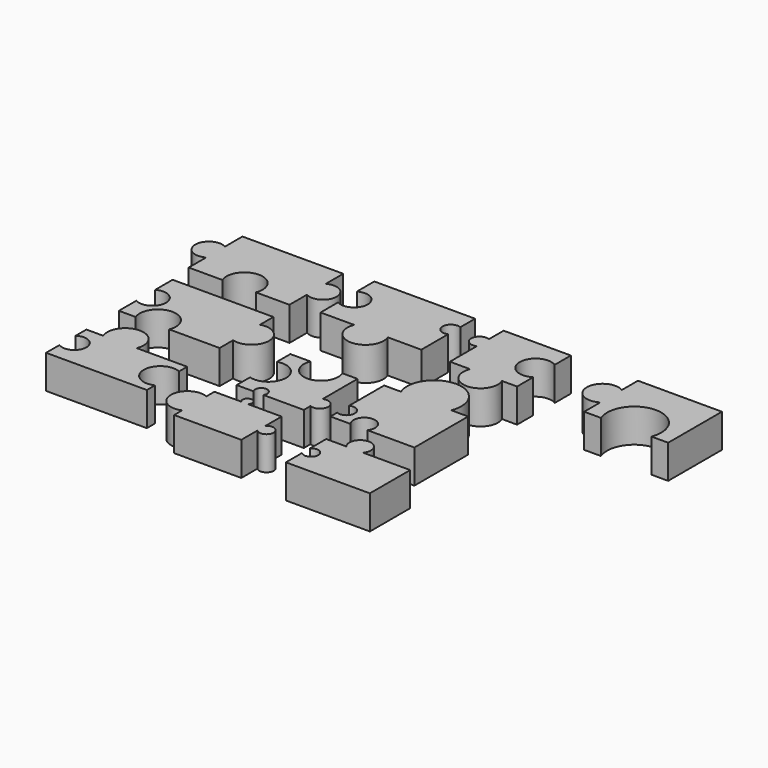
from build123d import *

# Parameters (mm, degrees)
F1_DEPTH  = 25.4
F3_DEPTH  = 25.4
F5_DEPTH  = 25.4
F7_DEPTH  = 25.4
F9_DEPTH  = 25.4
F11_DEPTH = 25.4
F13_DEPTH = 25.4
F15_DEPTH = 25.4
F17_DEPTH = 25.4
F19_DEPTH = 25.4


# Not quite as in the source:
# - a feature names something its author has since deleted; it is built from what else it names


with BuildPart() as f1:
    # F0 (on Top) → F1 (new body)
    with BuildSketch(Plane.XY):
        with BuildLine():
            Line((-78.5367997915, 29.1591999254), (-78.5367997915, 46.9391999254))
            ThreePointArc((-78.5367997915, 46.9391999254), (-93.8558671318, 38.0491999254), (-78.5367997915, 29.1591999254))
        make_face()
        with BuildLine():
            Line((-2.3367997915, 63.4491999254), (-78.5367997915, 63.4491999254))
            Line((-78.5367997915, 63.4491999254), (-78.5367997915, 46.9391999254))
            Line((-78.5367997915, 46.9391999254), (-78.5367997915, 29.1591999254))
            Line((-78.5367997915, 29.1591999254), (-78.5367997915, 12.6491999254))
            Line((-78.5367997915, 12.6491999254), (-53.1367997915, 12.6491999254))
            ThreePointArc((-53.1367997915, 12.6491999254), (-40.4367997915, 31.4075185355), (-27.7367997915, 12.6491999254))
            Line((-27.7367997915, 12.6491999254), (-2.3367997915, 12.6491999254))
            Line((-2.3367997915, 12.6491999254), (-2.3367997915, 29.1591999254))
            Line((-2.3367997915, 29.1591999254), (-2.3367997915, 46.9391999254))
            Line((-2.3367997915, 46.9391999254), (-2.3367997915, 63.4491999254))
        make_face()
        with BuildLine():
            ThreePointArc((-2.3367997915, 29.1591999254), (12.9822675489, 38.0491999254), (-2.3367997915, 46.9391999254))
            Line((-2.3367997915, 46.9391999254), (-2.3367997915, 29.1591999254))
        make_face()
    extrude(amount=F1_DEPTH)


with BuildPart() as f3:
    # F2 (on Top) → F3 (new body)
    with BuildSketch(Plane.XY):
        with BuildLine():
            Line((68.946869266, 16.4046303093), (43.546869266, 16.4046303093))
            ThreePointArc((43.546869266, 16.4046303093), (56.246869266, -2.3536883008), (68.946869266, 16.4046303093))
        make_face()
        with BuildLine():
            Line((94.346869266, 67.2046303093), (18.146869266, 67.2046303093))
            Line((18.146869266, 67.2046303093), (18.146869266, 50.6946303093))
            ThreePointArc((18.146869266, 50.6946303093), (33.4659366064, 41.8046303093), (18.146869266, 32.9146303093))
            Line((18.146869266, 32.9146303093), (18.146869266, 16.4046303093))
            Line((18.146869266, 16.4046303093), (43.546869266, 16.4046303093))
            Line((43.546869266, 16.4046303093), (68.946869266, 16.4046303093))
            Line((68.946869266, 16.4046303093), (94.346869266, 16.4046303093))
            Line((94.346869266, 16.4046303093), (94.346869266, 41.8046303093))
            ThreePointArc((94.346869266, 41.8046303093), (85.5528445619, 47.5196303093), (94.346869266, 53.2346303093))
            Line((94.346869266, 53.2346303093), (94.346869266, 67.2046303093))
        make_face()
    extrude(amount=F3_DEPTH)


with BuildPart() as f5:
    # F4 (on Top) → F5 (new body)
    with BuildSketch(Plane.XY):
        with BuildLine():
            Line((-50.8, -5.4863997316), (-76.2, -5.4863997316))
            Line((-76.2, -5.4863997316), (-76.2, -21.9963997316))
            ThreePointArc((-76.2, -21.9963997316), (-60.8809326597, -30.8863997316), (-76.2, -39.7763997316))
            Line((-76.2, -39.7763997316), (-76.2, -56.2863997316))
            Line((-76.2, -56.2863997316), (-63.5, -56.2863997316))
            ThreePointArc((-63.5, -56.2863997316), (-50.8, -37.5280811215), (-38.1, -56.2863997316))
            Line((-38.1, -56.2863997316), (0, -56.2863997316))
            Line((0, -56.2863997316), (0, -43.5863997316))
            Line((0, -43.5863997316), (0, -18.1863997316))
            Line((0, -18.1863997316), (0, -5.4863997316))
            Line((0, -5.4863997316), (-25.4, -5.4863997316))
            ThreePointArc((-25.4, -5.4863997316), (-38.1, -24.2447183418), (-50.8, -5.4863997316))
        make_face()
        with BuildLine():
            Line((-25.4, -5.4863997316), (-50.8, -5.4863997316))
            ThreePointArc((-50.8, -5.4863997316), (-38.1, -24.2447183418), (-25.4, -5.4863997316))
        make_face()
        with BuildLine():
            ThreePointArc((0, -43.5863997316), (17.0691892663, -30.8863997316), (0, -18.1863997316))
            Line((0, -18.1863997316), (0, -43.5863997316))
        make_face()
    extrude(amount=F5_DEPTH)


with BuildPart() as f7:
    # F6 (on Top) → F7 (new body)
    with BuildSketch(Plane.XY):
        with BuildLine():
            ThreePointArc((88.2271643072, -80.6943764091), (97.0211890114, -74.9793764091), (88.2271643072, -69.2643764091))
            Line((88.2271643072, -69.2643764091), (88.2271643072, -80.6943764091))
        make_face()
        with BuildLine():
            Line((52.6671643072, -36.2443764091), (37.4271643072, -36.2443764091))
            Line((37.4271643072, -36.2443764091), (37.4271643072, -48.9443764091))
            ThreePointArc((37.4271643072, -48.9443764091), (54.4963535736, -61.6443764091), (37.4271643072, -74.3443764091))
            Line((37.4271643072, -74.3443764091), (37.4271643072, -87.0443764091))
            Line((37.4271643072, -87.0443764091), (50.1271643072, -87.0443764091))
            ThreePointArc((50.1271643072, -87.0443764091), (53.9371643072, -79.9253262892), (57.7471643072, -87.0443764091))
            Line((57.7471643072, -87.0443764091), (88.2271643072, -87.0443764091))
            Line((88.2271643072, -87.0443764091), (88.2271643072, -80.6943764091))
            Line((88.2271643072, -80.6943764091), (88.2271643072, -69.2643764091))
            Line((88.2271643072, -69.2643764091), (88.2271643072, -36.2443764091))
            Line((88.2271643072, -36.2443764091), (76.7971643072, -36.2443764091))
            ThreePointArc((76.7971643072, -36.2443764091), (64.7321643072, -54.4152367704), (52.6671643072, -36.2443764091))
        make_face()
    extrude(amount=F7_DEPTH)


with BuildPart() as f9:
    # F8 (on Top) → F9 (new body)
    with BuildSketch(Plane.XY):
        with BuildLine():
            Line((117.092727313, 40.3700199814), (117.092727313, 14.9700199814))
            Line((117.092727313, 14.9700199814), (132.332727313, 14.9700199814))
            Line((132.332727313, 14.9700199814), (156.462727313, 14.9700199814))
            Line((156.462727313, 14.9700199814), (167.892727313, 14.9700199814))
            Line((167.892727313, 14.9700199814), (167.892727313, 30.2100199814))
            ThreePointArc((167.892727313, 30.2100199814), (149.5615712753, 40.3700199814), (167.892727313, 50.5300199814))
            Line((167.892727313, 50.5300199814), (167.892727313, 65.7700199814))
            Line((167.892727313, 65.7700199814), (117.092727313, 65.7700199814))
            Line((117.092727313, 65.7700199814), (117.092727313, 51.8000199814))
            Line((117.092727313, 51.8000199814), (117.092727313, 40.3700199814))
        make_face()
        with BuildLine():
            Line((156.462727313, 14.9700199814), (132.332727313, 14.9700199814))
            ThreePointArc((132.332727313, 14.9700199814), (144.397727313, -3.2008403799), (156.462727313, 14.9700199814))
        make_face()
        with BuildLine():
            ThreePointArc((117.092727313, 51.8000199814), (108.2987026089, 46.0850199814), (117.092727313, 40.3700199814))
            Line((117.092727313, 40.3700199814), (117.092727313, 51.8000199814))
        make_face()
    extrude(amount=F9_DEPTH)


with BuildPart() as f11:
    # F10 (on Top) → F11 (new body)
    with BuildSketch(Plane.XY):
        with BuildLine():
            Line((218.9528409719, 29.8046059906), (218.9528409719, 50.1246059906))
            ThreePointArc((218.9528409719, 50.1246059906), (200.6216849342, 39.9646059906), (218.9528409719, 29.8046059906))
        make_face()
        with BuildLine():
            Line((282.4528409719, 65.3646059906), (218.9528409719, 65.3646059906))
            Line((218.9528409719, 65.3646059906), (218.9528409719, 50.1246059906))
            Line((218.9528409719, 50.1246059906), (218.9528409719, 29.8046059906))
            Line((218.9528409719, 29.8046059906), (218.9528409719, 14.5646059906))
            Line((218.9528409719, 14.5646059906), (231.6528409719, 14.5646059906))
            ThreePointArc((231.6528409719, 14.5646059906), (250.7028409719, 42.7020839058), (269.7528409719, 14.5646059906))
            Line((269.7528409719, 14.5646059906), (282.4528409719, 14.5646059906))
            Line((282.4528409719, 14.5646059906), (282.4528409719, 65.3646059906))
        make_face()
    extrude(amount=F11_DEPTH)


with BuildPart() as f13:
    # F12 (on Top) → F13 (new body)
    with BuildSketch(Plane.XY):
        with BuildLine():
            ThreePointArc((156.5685857674, -33.0217852473), (137.5185857674, -4.8843073321), (118.4685857674, -33.0217852473))
            Line((118.4685857674, -33.0217852473), (156.5685857674, -33.0217852473))
        make_face()
        with BuildLine():
            Line((118.4685857674, -33.0217852473), (105.7685857674, -33.0217852473))
            Line((105.7685857674, -33.0217852473), (105.7685857674, -66.0417852473))
            ThreePointArc((105.7685857674, -66.0417852473), (114.5626104715, -71.7567852473), (105.7685857674, -77.4717852473))
            Line((105.7685857674, -77.4717852473), (105.7685857674, -83.8217852473))
            Line((105.7685857674, -83.8217852473), (121.0085857674, -83.8217852473))
            ThreePointArc((121.0085857674, -83.8217852473), (127.3585857674, -70.6098174658), (133.7085857674, -83.8217852473))
            Line((133.7085857674, -83.8217852473), (169.2685857674, -83.8217852473))
            Line((169.2685857674, -83.8217852473), (169.2685857674, -33.0217852473))
            Line((169.2685857674, -33.0217852473), (156.5685857674, -33.0217852473))
            Line((156.5685857674, -33.0217852473), (118.4685857674, -33.0217852473))
        make_face()
    extrude(amount=F13_DEPTH)


with BuildPart() as f15:
    # F14 (on Top) → F15 (new body)
    with BuildSketch(Plane.XY):
        with BuildLine():
            ThreePointArc((-38.1, -86.9720183969), (-50.8, -68.2136997867), (-63.5, -86.9720183969))
            Line((-63.5, -86.9720183969), (-38.1, -86.9720183969))
        make_face()
        with BuildLine():
            Line((-63.5, -86.9720183969), (-76.2, -86.9720183969))
            Line((-76.2, -86.9720183969), (-76.2, -97.1320183969))
            ThreePointArc((-76.2, -97.1320183969), (-61.9618997603, -104.7520183969), (-76.2, -112.3720183969))
            Line((-76.2, -112.3720183969), (-76.2, -125.0720183969))
            Line((-76.2, -125.0720183969), (0, -125.0720183969))
            Line((0, -125.0720183969), (0, -117.4520183969))
            ThreePointArc((0, -117.4520183969), (-17.5880494083, -106.0220183969), (0, -94.5920183969))
            Line((0, -94.5920183969), (0, -86.9720183969))
            Line((0, -86.9720183969), (-38.1, -86.9720183969))
            Line((-38.1, -86.9720183969), (-63.5, -86.9720183969))
        make_face()
    extrude(amount=F15_DEPTH)


with BuildPart() as f17:
    # F16 (on Top) → F17 (new body)
    with BuildSketch(Plane.XY):
        Polygon((52.8417903644, -101.8752300191), (32.5217903644, -101.8752300191), (32.5217903644, -109.4952300191), (32.5217903644, -132.3552300191), (32.5217903644, -139.9752300191), (83.3217903644, -139.9752300191), (83.3217903644, -124.7352300191), (83.3217903644, -117.1152300191), (83.3217903644, -101.8752300191), (57.9217903644, -101.8752300191), align=None)
        with BuildLine():
            ThreePointArc((57.9217903644, -101.8752300191), (55.3817903644, -95.7431275707), (52.8417903644, -101.8752300191))
            Line((52.8417903644, -101.8752300191), (57.9217903644, -101.8752300191))
        make_face()
        with BuildLine():
            Line((32.5217903644, -132.3552300191), (32.5217903644, -109.4952300191))
            ThreePointArc((32.5217903644, -109.4952300191), (14.9337409561, -120.9252300191), (32.5217903644, -132.3552300191))
        make_face()
        with BuildLine():
            ThreePointArc((83.3217903644, -124.7352300191), (92.519944037, -120.9252300191), (83.3217903644, -117.1152300191))
            Line((83.3217903644, -117.1152300191), (83.3217903644, -124.7352300191))
        make_face()
    extrude(amount=F17_DEPTH)


with BuildPart() as f19:
    # F18 (on Top) → F19 (new body)
    with BuildSketch(Plane.XY):
        with BuildLine():
            ThreePointArc((149.7844299936, -107.8747646904), (143.4344299936, -94.6627969089), (137.0844299936, -107.8747646904))
            Line((137.0844299936, -107.8747646904), (149.7844299936, -107.8747646904))
        make_face()
        with BuildLine():
            Line((137.0844299936, -107.8747646904), (121.8444299936, -107.8747646904))
            Line((121.8444299936, -107.8747646904), (121.8444299936, -123.1147646904))
            ThreePointArc((121.8444299936, -123.1147646904), (131.0425836663, -126.9247646904), (121.8444299936, -130.7347646904))
            Line((121.8444299936, -130.7347646904), (121.8444299936, -145.9747646904))
            Line((121.8444299936, -145.9747646904), (185.3444299936, -145.9747646904))
            Line((185.3444299936, -145.9747646904), (185.3444299936, -107.8747646904))
            Line((185.3444299936, -107.8747646904), (149.7844299936, -107.8747646904))
            Line((149.7844299936, -107.8747646904), (137.0844299936, -107.8747646904))
        make_face()
    extrude(amount=F19_DEPTH)


solid = Compound([f1.part, f3.part, f5.part, f7.part, f9.part, f11.part, f13.part, f15.part, f17.part, f19.part])
